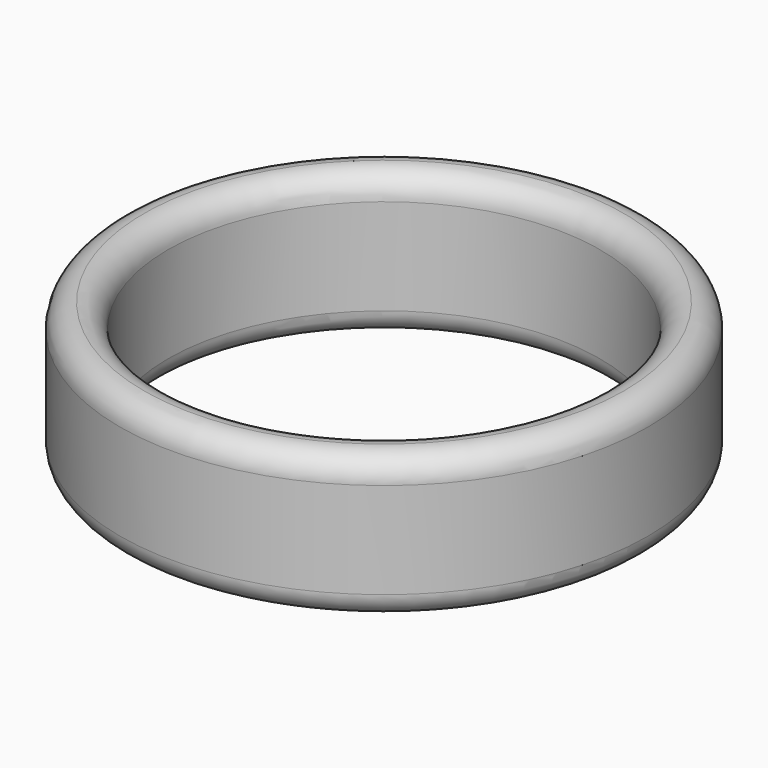
from build123d import *

# Parameters (mm, degrees)
F0_R     = 11
F0_R_2   = 9
F1_DEPTH = 6
F2_R     = 0.99999


# Not quite as in the source:
# - a fillet or chamfer is up to 0.001 mm smaller than in the source, because OpenCascade refuses the exact size


with BuildPart() as f1:
    # F0 (on Top) → F1 (new body)
    with BuildSketch(Plane.XY):
        Circle(F0_R)
        Circle(F0_R_2, mode=Mode.SUBTRACT)
    extrude(amount=F1_DEPTH)

    # F2 (radius 1 in the source; OpenCascade refuses exactly that, so slightly less here)
    f2_edges = [f1.edges().sort_by_distance(p)[0] for p in [
        (-9, 0, 6),
        (-9, 0, 0),
        (-11, 0, 6),
        (-11, 0, 0),
    ]]
    fillet(f2_edges, radius=F2_R)


solid = f1.part
